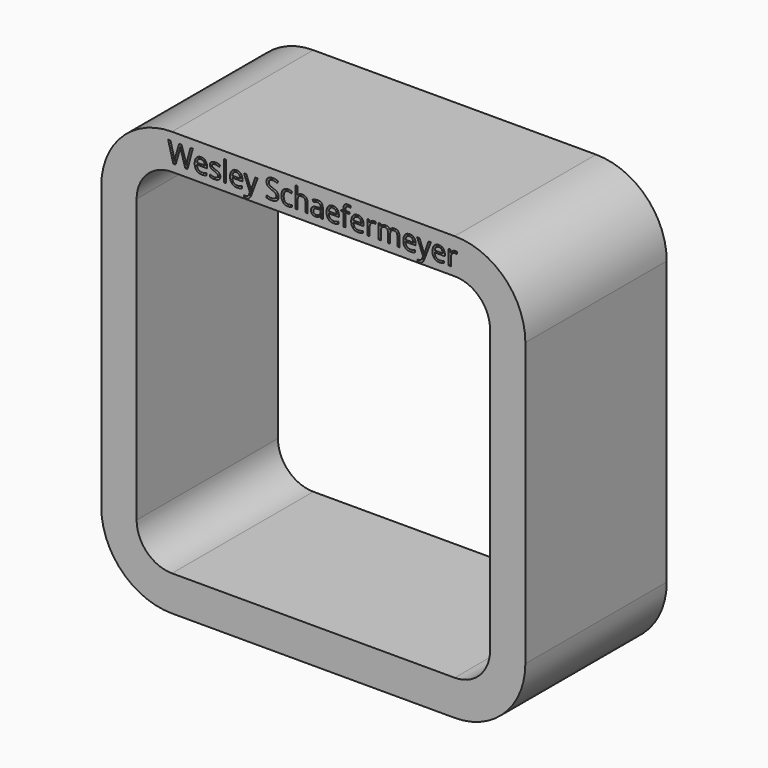
from build123d import *

# Parameters (mm, degrees)
F1_DEPTH     = 50
F2_TEXT_SIZE = 7.7553766055
F3_DEPTH     = 1.5


# Not quite as in the source:
# - Text() gives the source's letters only with a copy of the font that has no kerning and outlines rounded to 1/6400 em; it was checked with that copy


with BuildPart() as f1:
    # F0 (on Front) → F1 (new body)
    with BuildSketch(Plane.XZ):
        with BuildLine():
            Line((40, 60), (-40, 60))
            ThreePointArc((-40, 60), (-54.1421356237, 54.1421356237), (-60, 40))
            Line((-60, 40), (-60, -40))
            ThreePointArc((-60, -40), (-54.1421356237, -54.1421356237), (-40, -60))
            Line((-40, -60), (40, -60))
            ThreePointArc((40, -60), (54.1421356237, -54.1421356237), (60, -40))
            Line((60, -40), (60, 40))
            ThreePointArc((60, 40), (54.1421356237, 54.1421356237), (40, 60))
        make_face()
        with BuildLine():
            Line((-40, 50), (40, 50))
            ThreePointArc((40, 50), (47.0710678119, 47.0710678119), (50, 40))
            Line((50, 40), (50, -40))
            ThreePointArc((50, -40), (47.0710678119, -47.0710678119), (40, -50))
            Line((40, -50), (-40, -50))
            ThreePointArc((-40, -50), (-47.0710678119, -47.0710678119), (-50, -40))
            Line((-50, -40), (-50, 40))
            ThreePointArc((-50, 40), (-47.0710678119, 47.0710678119), (-40, 50))
        make_face(mode=Mode.SUBTRACT)
    extrude(amount=F1_DEPTH)

    # F2 (on face) → F3 (cut)
    with BuildSketch(Plane.XZ.offset(50)):
        with Locations((-41.1862, 52.1344952285)):
            Text('Wesley Schaefermeyer', F2_TEXT_SIZE, font='Open Sans', text_align=(TextAlign.LEFT, TextAlign.BOTTOM))
    extrude(amount=-F3_DEPTH, mode=Mode.SUBTRACT)


solid = f1.part
